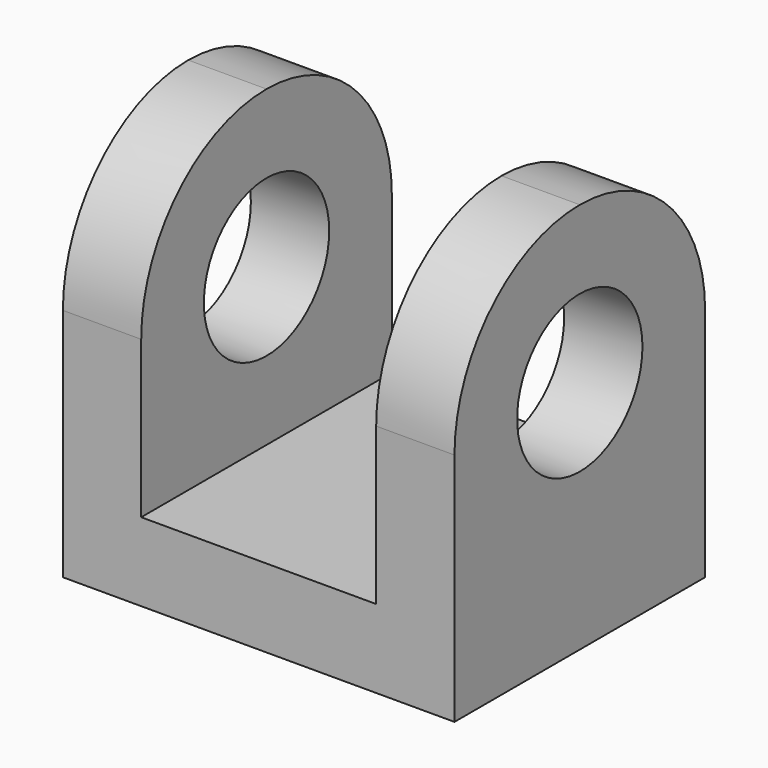
from build123d import *

# Parameters (mm, degrees)
F0_W     = 5
F0_H     = 4
F1_DEPTH = 5
F2_R     = 1.99999
F3_R     = 1
F4_DEPTH = 25
F7_W     = 3
F7_H     = 4
F8_DEPTH = 4


# Not quite as in the source:
# - a fillet or chamfer is up to 0.001 mm smaller than in the source, because OpenCascade refuses the exact size


with BuildPart() as f1:
    # F0 (on Top) → F1 (new body)
    with BuildSketch(Plane.XY):
        with Locations((2.5, 2)):
            Rectangle(F0_W, F0_H)
    extrude(amount=F1_DEPTH)

    # F2 (radius 2 in the source; OpenCascade refuses exactly that, so slightly less here)
    f2_edges = [f1.edges().sort_by_distance(p)[0] for p in [
        (2.5, 0, 5),
        (2.5, 4, 5),
    ]]
    fillet(f2_edges, radius=F2_R)

    # F3 (on face) → F4 (cut)
    with BuildSketch(Plane.YZ.offset(5)):
        with Locations((2, 3)):
            Circle(F3_R)
    extrude(amount=-F4_DEPTH, mode=Mode.SUBTRACT)

    # F7 (on face) → F8 (cut)
    with BuildSketch(Plane.XY.offset(5)):
        with Locations((2.5, 2)):
            Rectangle(F7_W, F7_H)
    extrude(amount=-F8_DEPTH, mode=Mode.SUBTRACT)


solid = f1.part
